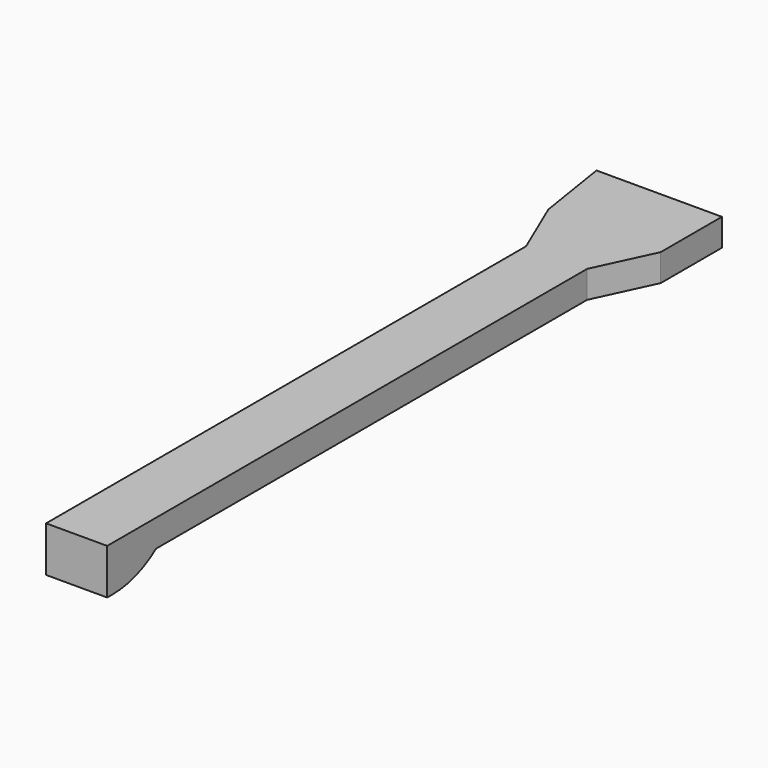
from build123d import *

# Parameters (mm, degrees)
F0_W        = 17.0710533857
F0_H        = 167.5858162344
F1_DEPTH    = 7.62
F2_W        = 17.0710533857
F2_H        = 17.0666188933
F3_DEPTH    = 5.08
F4_T1_DEPTH = 92.8391963602


# Not quite as in the source:
# - a fillet or chamfer that OpenCascade refuses, or shapes differently, is made with other operations: its cross-section is extruded or revolved along the edge and cut away or added


with BuildPart() as f1:
    # F0 (on Top) → F1 (new body)
    with BuildSketch(Plane.XY):
        with Locations((-152.5016650558, 70.9913838655)):
            Rectangle(F0_W, F0_H)
        Polygon((-168.1138426065, 171.4205145836), (-161.0371917486, 154.7842919827), (-143.9661383629, 154.7842919827), (-136.3786160946, 170.9794849157), (-136.3786160946, 192.3550665379), (-171.417593956, 192.3550665379), align=None)
    extrude(amount=F1_DEPTH)

    # F2 (on face) → F3 (join)
    with BuildSketch(Plane(origin=(0, 0, 0), x_dir=(1, 0, 0), z_dir=(0, 0, -1))):
        with Locations((-152.5016650558, 4.2682148051)):
            Rectangle(F2_W, F2_H)
    extrude(amount=F3_DEPTH)

    # F4: fillet of radius 25.1416200386 on 1 edges, made by hand

    # F4_s2 → F4_t1 (cut)
    with BuildSketch(Plane.YZ.offset(-198.9212632358)):
        with BuildLine():
            ThreePointArc((4.2650946416, 0), (-2.8973065821, -3.7761932686), (-10.8885339533, -5.08))
            Line((-10.8885339533, -5.08), (-10.8885339533, -5.5828324008))
            Line((-10.8885339533, -5.5828324008), (4.2650946416, -5.5828324008))
            Line((4.2650946416, -5.5828324008), (4.7679270424, -5.08))
            ThreePointArc((4.7679270424, -5.08), (4.7679270424, -2.54), (4.5681672135, -0.4012324008))
            Line((4.5681672135, -0.4012324008), (4.2650946416, 0))
        make_face()
    extrude(amount=F4_T1_DEPTH, mode=Mode.SUBTRACT)


solid = f1.part
